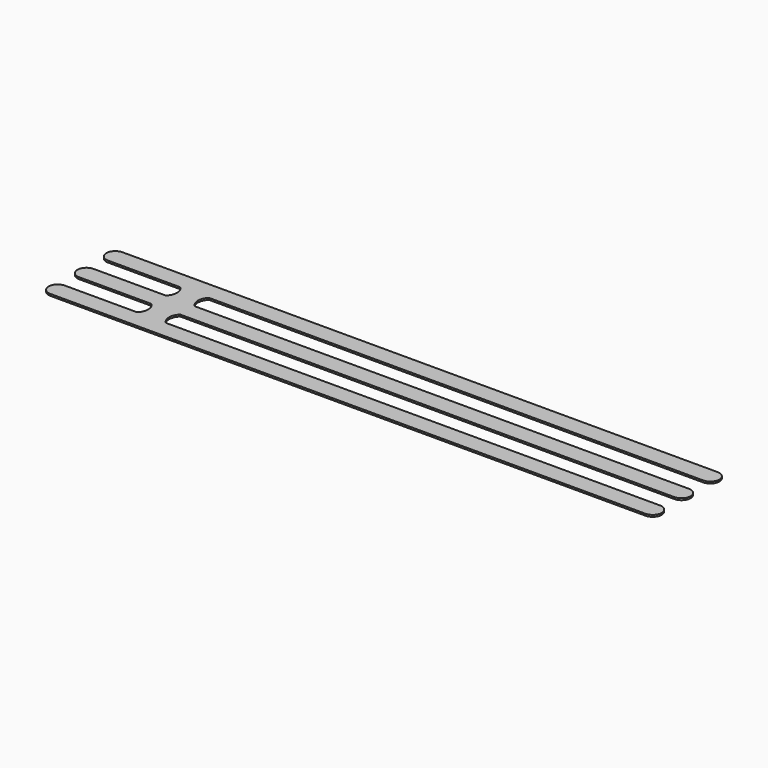
from build123d import *

# Parameters (mm, degrees)
F1_DEPTH = 0.635


# Not quite as in the source:
# - a feature names something its author has since deleted; it is built from what else it names


with BuildPart() as f1:
    # F0 (on Top) → F1 (new body)
    with BuildSketch(Plane.XY):
        with BuildLine():
            ThreePointArc((107.95, 0), (107.0200640303, 2.2450640303), (104.775, 3.175))
            Line((104.775, 3.175), (-69.215, 3.175))
            Line((-69.215, 3.175), (-74.295, 3.175))
            Line((-74.295, 3.175), (-74.295, -3.175))
            Line((-74.295, -3.175), (-69.215, -3.175))
            Line((-69.215, -3.175), (104.775, -3.175))
            ThreePointArc((104.775, -3.175), (107.0200640303, -2.2450640303), (107.95, 0))
        make_face()
        with BuildLine():
            Line((-74.295, -3.175), (-74.295, 3.175))
            Line((-74.295, 3.175), (-79.375, 3.175))
            Line((-79.375, 3.175), (-104.775, 3.175))
            ThreePointArc((-104.775, 3.175), (-107.0200640303, 2.2450640303), (-107.95, 0))
            ThreePointArc((-107.95, 0), (-107.0200640303, -2.2450640303), (-104.775, -3.175))
            Line((-104.775, -3.175), (-79.375, -3.175))
            Line((-79.375, -3.175), (-74.295, -3.175))
        make_face()
        with BuildLine():
            Line((-74.295, 9.525), (-69.215, 9.525))
            Line((-69.215, 9.525), (104.775, 9.525))
            ThreePointArc((104.775, 9.525), (107.0200640303, 10.4549359697), (107.95, 12.7))
            ThreePointArc((107.95, 12.7), (107.0200640302, 14.9450640302), (104.775, 15.875))
            Line((104.775, 15.875), (-74.295, 15.875))
            Line((-74.295, 15.875), (-74.295, 9.525))
        make_face()
        with BuildLine():
            Line((-79.375, 9.525), (-74.295, 9.525))
            Line((-74.295, 9.525), (-74.295, 15.875))
            Line((-74.295, 15.875), (-104.775, 15.875))
            ThreePointArc((-104.775, 15.875), (-107.0200640302, 14.9450640302), (-107.95, 12.7))
            ThreePointArc((-107.95, 12.7), (-107.0200640303, 10.4549359697), (-104.775, 9.525))
            Line((-104.775, 9.525), (-79.375, 9.525))
        make_face()
        with BuildLine():
            Line((-69.2150000001, -9.5250000001), (-74.295, -9.5250000001))
            Line((-74.295, -9.5250000001), (-74.295, -15.875))
            Line((-74.295, -15.875), (104.775, -15.875))
            ThreePointArc((104.775, -15.875), (107.0200640302, -14.9450640302), (107.95, -12.7))
            ThreePointArc((107.95, -12.7), (107.0200640303, -10.4549359697), (104.775, -9.525))
            Line((104.775, -9.5250000001), (-69.2150000001, -9.5250000001))
        make_face()
        with BuildLine():
            Line((-74.295, -15.875), (-74.295, -9.5250000001))
            Line((-74.295, -9.5250000001), (-79.375, -9.5250000001))
            Line((-79.375, -9.5250000001), (-104.775, -9.5250000001))
            ThreePointArc((-104.775, -9.525), (-107.0200640303, -10.4549359697), (-107.95, -12.7))
            ThreePointArc((-107.95, -12.7), (-107.0200640302, -14.9450640302), (-104.775, -15.875))
            Line((-104.775, -15.875), (-74.295, -15.875))
        make_face()
        with BuildLine():
            Line((-79.375, 3.175), (-74.295, 3.175))
            Line((-74.295, 3.175), (-74.295, 9.525))
            Line((-74.295, 9.525), (-79.375, 9.525))
            ThreePointArc((-79.375, 9.525), (-77.98351653, 6.35), (-79.375, 3.175))
        make_face()
        with BuildLine():
            Line((-74.295, 3.175), (-69.215, 3.175))
            ThreePointArc((-69.215, 3.175), (-70.6064834701, 6.35), (-69.215, 9.525))
            Line((-69.215, 9.525), (-74.295, 9.525))
            Line((-74.295, 9.525), (-74.295, 3.175))
        make_face()
        with BuildLine():
            Line((-74.295, -9.5250000001), (-74.295, -3.175))
            Line((-74.295, -3.175), (-79.375, -3.175))
            ThreePointArc((-79.375, -3.175), (-77.9835165299, -6.35), (-79.375, -9.525))
            Line((-79.375, -9.5250000001), (-74.295, -9.5250000001))
        make_face()
        with BuildLine():
            Line((-69.215, -3.175), (-74.295, -3.175))
            Line((-74.295, -3.175), (-74.295, -9.5250000001))
            Line((-74.295, -9.5250000001), (-69.2150000001, -9.5250000001))
            ThreePointArc((-69.2150000001, -9.525), (-70.6064834702, -6.35), (-69.215, -3.175))
        make_face()
    extrude(amount=F1_DEPTH)


solid = f1.part
